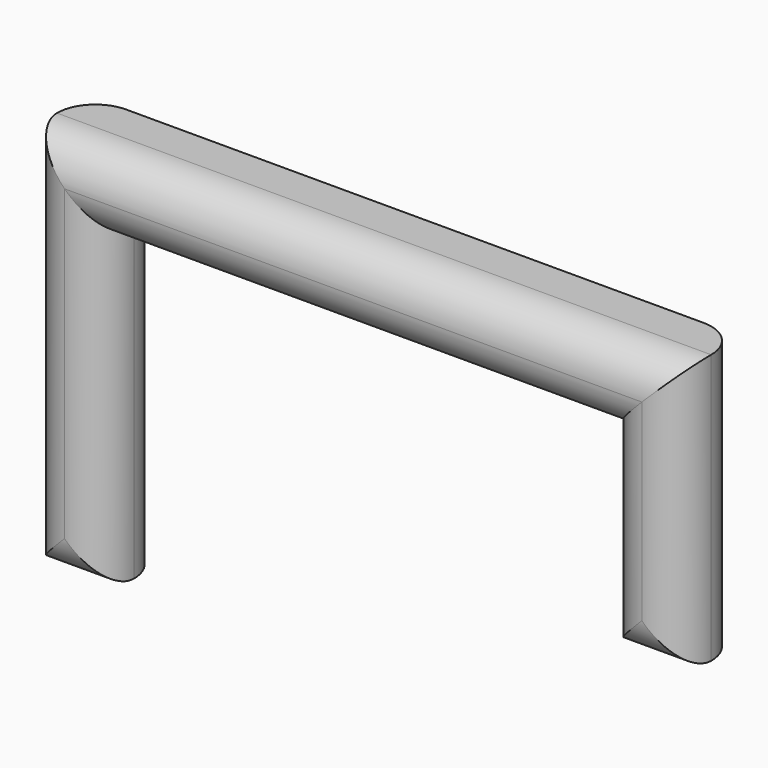
from build123d import *

# Parameters (mm, degrees)
F0_W     = 10
F0_H     = 10
F1_DEPTH = 50
F2_W     = 10
F2_H     = 10
F3_DEPTH = 75
F4_W     = 10
F4_H     = 10
F5_DEPTH = 25
F6_R     = 4.99999


# Not quite as in the source:
# - a fillet or chamfer is up to 0.001 mm smaller than in the source, because OpenCascade refuses the exact size


with BuildPart() as f1:
    # F0 (on Top) → F1 (new body)
    with BuildSketch(Plane.XY):
        with Locations((5, 5)):
            Rectangle(F0_W, F0_H)
    extrude(amount=F1_DEPTH)

    # F2 (on face) → F3 (join)
    with BuildSketch(Plane.YZ.offset(10)):
        with Locations((5, 45)):
            Rectangle(F2_W, F2_H)
    extrude(amount=F3_DEPTH)

    # F4 (on face) → F5 (join)
    with BuildSketch(Plane(origin=(0, 0, 40), x_dir=(1, 0, 0), z_dir=(0, 0, -1))):
        with Locations((80, -5)):
            Rectangle(F4_W, F4_H)
    extrude(amount=F5_DEPTH)

    # F6 (radius 5 in the source; OpenCascade refuses exactly that, so slightly less here)
    f6_edges = [f1.edges().sort_by_distance(p)[0] for p in [
        (10, 0, 20),
        (0, 0, 25),
        (0, 10, 25),
        (10, 10, 20),
        (42.5, 0, 50),
        (42.5, 0, 40),
        (42.5, 10, 40),
        (85, 0, 32.5),
        (80, 0, 15),
        (75, 0, 27.5),
        (5, 0, 0),
        (85, 10, 32.5),
        (75, 10, 27.5),
    ]]
    fillet(f6_edges, radius=F6_R)


solid = f1.part
